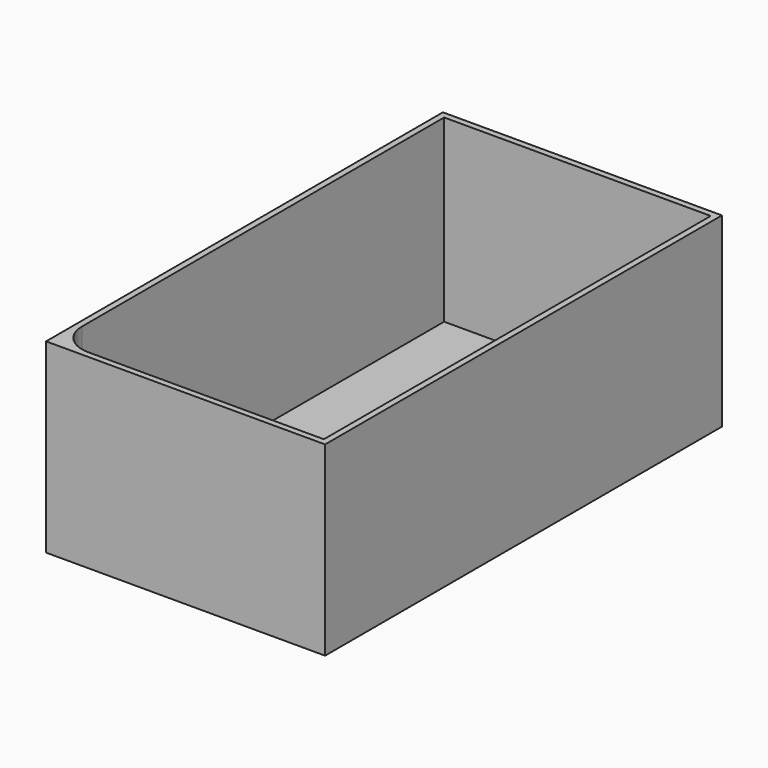
from build123d import *

# Parameters (mm, degrees)
F0_W     = 114.3
F0_H     = 203.2
F1_DEPTH = 76.2
F2_T     = -2.54
F3_R     = 12.7


with BuildPart() as f1:
    # F0 (on Top) → F1 (new body)
    with BuildSketch(Plane.XY):
        with Locations((0, 38.1)):
            Rectangle(F0_W, F0_H)
    extrude(amount=F1_DEPTH)

    # F2
    f2_openings = [f1.faces().sort_by_distance(p)[0] for p in [
        (0, 38.1, 76.2),
    ]]
    offset(amount=F2_T, openings=f2_openings)

    # F3
    f3_edges = [f1.edges().sort_by_distance(p)[0] for p in [
        (-54.61, -60.96, 39.37),
    ]]
    fillet(f3_edges, radius=F3_R)


solid = f1.part
